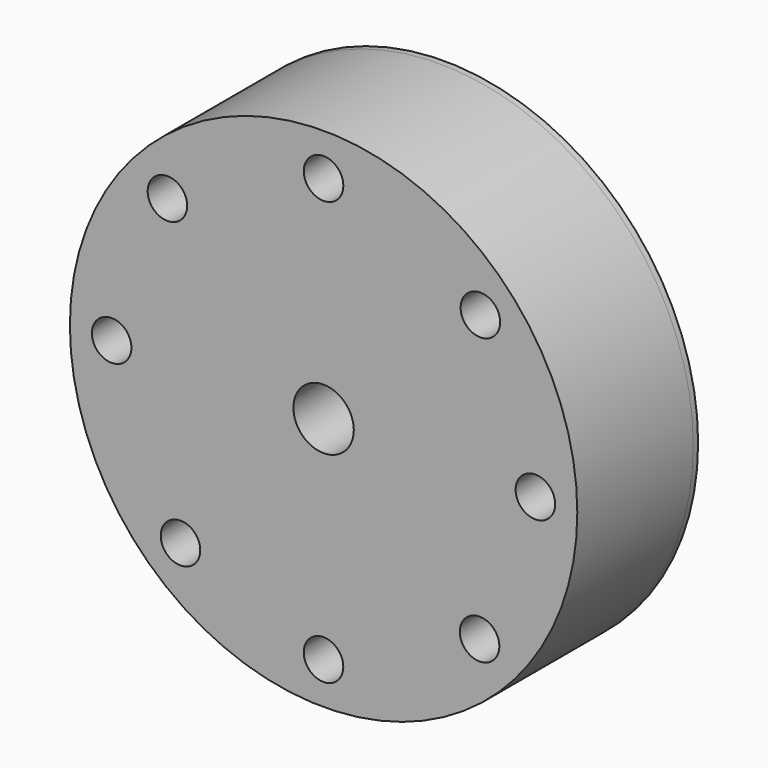
from build123d import *

# Parameters (mm, degrees)
F0_R     = 42
F0_R_2   = 3.2723941489
F0_R_3   = 15
F0_R_4   = 8.75
F1_DEPTH = 25
F0_R_5   = 5
F2_DEPTH = 25
F7_DEPTH = 24


# Not quite as in the source:
# - the program builds the solid bodies; features that only make, move or delete a surface that nothing else refers to are left out


with BuildPart() as f1:
    # F0 (on Front) → F1 (new body)
    with BuildSketch(Plane.XZ):
        Circle(F0_R)
        with Locations((-23.6904930325, -25.7949024873)):
            Circle(F0_R_2, mode=Mode.SUBTRACT)
        with Locations((-0.0140495196, -35.0812149592)):
            Circle(F0_R_2, mode=Mode.SUBTRACT)
        with Locations((25.8215879073, -23.6839220737)):
            Circle(F0_R_2, mode=Mode.SUBTRACT)
        with Locations((-35.0852801235, 0.0172716529)):
            Circle(F0_R_2, mode=Mode.SUBTRACT)
        with Locations((-25.8480679978, 23.7130210266)):
            Circle(F0_R_2, mode=Mode.SUBTRACT)
        with Locations((-0.0057062035, 35.0350632497)):
            Circle(F0_R_2, mode=Mode.SUBTRACT)
        Circle(F0_R_3, mode=Mode.SUBTRACT)
        with Locations((35.0598417296, 0.0224386821)):
            Circle(F0_R_2, mode=Mode.SUBTRACT)
        with Locations((25.9556279527, 23.5858062447)):
            Circle(F0_R_2, mode=Mode.SUBTRACT)
        Circle(F0_R_3)
        Circle(F0_R_4, mode=Mode.SUBTRACT)
    extrude(amount=F1_DEPTH)

    # F0 (on Front) → F2 (join)
    with BuildSketch(Plane.XZ):
        Circle(F0_R_4)
        Circle(F0_R_5, mode=Mode.SUBTRACT)
    extrude(amount=F2_DEPTH)

    # F7 (add): a face of the model
    f7_faces = [f1.faces().sort_by_distance(p)[0] for p in [
        (-40.8120606076, -25, 0),
    ]]
    extrude(f7_faces, amount=-F7_DEPTH)


solid = f1.part
